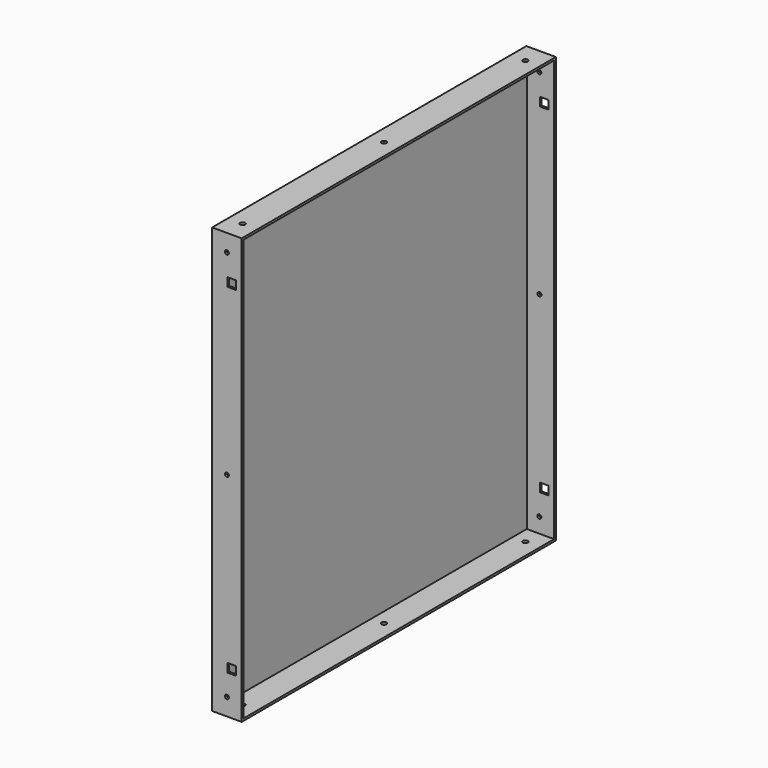
from build123d import *

# Parameters (mm, degrees)
F0_W     = 38.1
F0_H     = 506.73
F1_DEPTH = 274.6375
F2_T     = -2.778125
F3_R     = 2.5796875
F3_W     = 11.1125
F3_H     = 11.1125
F4_DEPTH = 506.731
F5_R     = 3.175
F6_DEPTH = 549.276


# Not quite as in the source:
# - a feature names something its author has since deleted; it is built from what else it names


with BuildPart() as f1:
    # F0 (on Top) → F1 (new body, symmetric)
    with BuildSketch(Plane.XY):
        with Locations((19.05, 253.365)):
            Rectangle(F0_W, F0_H)
    extrude(amount=F1_DEPTH, both=True)

    # F2
    f2_openings = [f1.faces().sort_by_distance(p)[0] for p in [
        (38.1, 253.365, 0),
    ]]
    offset(amount=F2_T, openings=f2_openings)

    # F3 (on face) → F4 (cut, through all)
    with BuildSketch(Plane(origin=(0, 506.73, 0), x_dir=(-1, 0, 0), z_dir=(0, 1, 0))):
        with Locations((-19.05, 252.4125)):
            Circle(F3_R)
        with Locations((-19.05, 0)):
            Circle(F3_R)
        with Locations((-19.05, -252.4125)):
            Circle(F3_R)
        with Locations((-25.4, 219.075)):
            Rectangle(F3_W, F3_H)
        with Locations((-25.4, -219.075)):
            Rectangle(F3_W, F3_H)
    extrude(amount=-F4_DEPTH, mode=Mode.SUBTRACT)

    # F5 (on face) → F6 (cut, through all)
    with BuildSketch(Plane.XY.offset(274.6375)):
        with Locations((19.05, 481.33)):
            Circle(F5_R)
        with Locations((19.05, 253.365)):
            Circle(F5_R)
        with Locations((19.05, 25.4)):
            Circle(F5_R)
    extrude(amount=-F6_DEPTH, mode=Mode.SUBTRACT)


solid = f1.part
